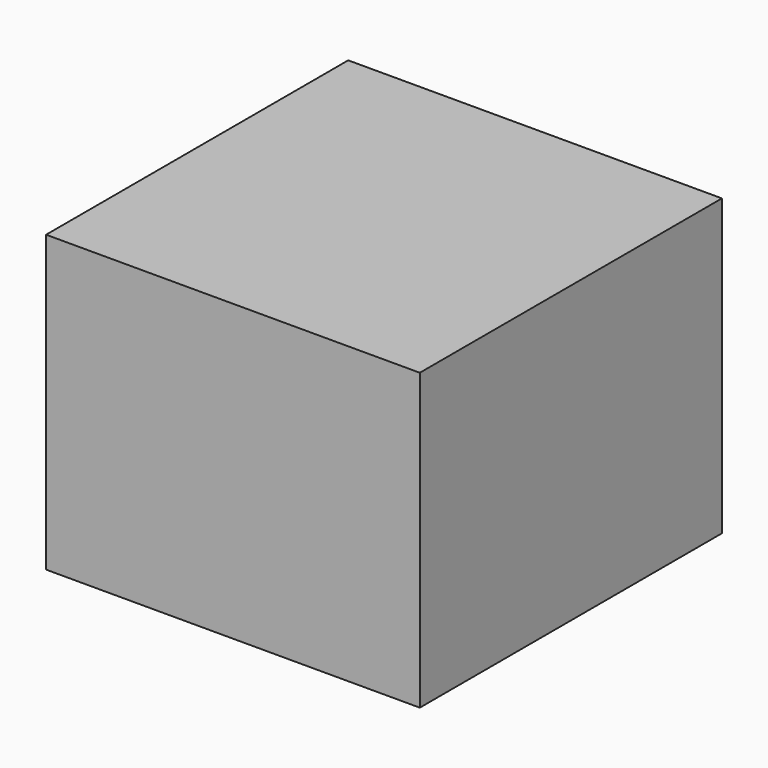
from build123d import *

# Parameters (mm, degrees)
F0_W     = 67.9279565811
F0_H     = 88.0647003651
F1_DEPTH = 53.594
F2_W     = 67.9279565811
F2_H     = 19.4227546453
F3_DEPTH = 89.662


# Not quite as in the source:
# - a feature of the source that left no trace in its solid (it failed there, or was rolled back) is left out


with BuildPart() as f1:
    # F0 (on Top) → F1 (new body)
    with BuildSketch(Plane.XY):
        Rectangle(F0_W, F0_H)
    extrude(amount=F1_DEPTH)

    # F2 (on face) → F3 (cut)
    with BuildSketch(Plane.XY.offset(53.594)):
        with Locations((0, -34.3209728599)):
            Rectangle(F2_W, F2_H)
    extrude(amount=-F3_DEPTH, mode=Mode.SUBTRACT)


solid = f1.part
